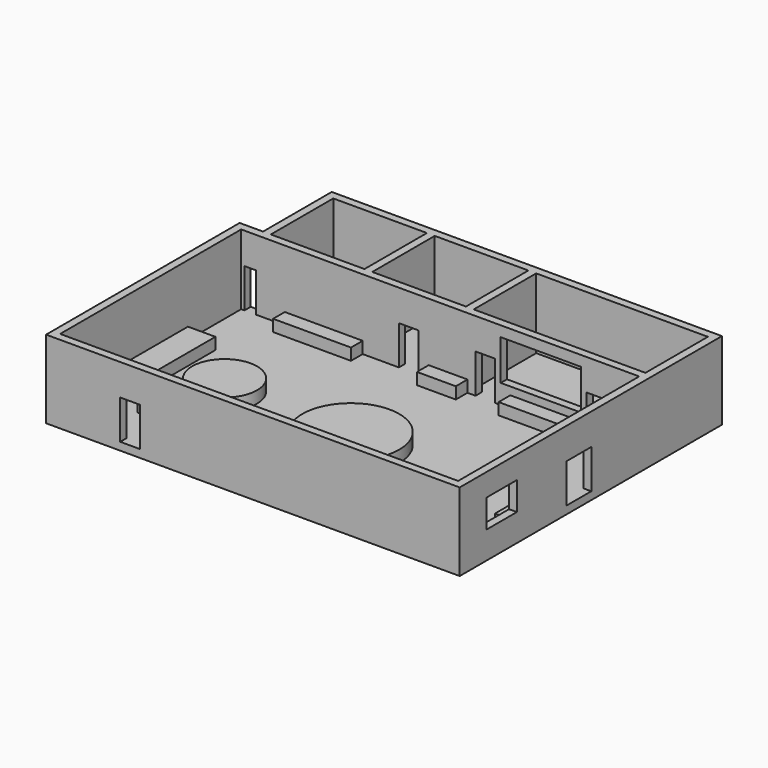
from build123d import *

# Parameters (mm, degrees)
F0_W      = 1346.2
F0_H      = 787.4
F1_DEPTH  = 254
F2_T      = -25.4
F3_W      = 1270
F3_H      = 254
F4_DEPTH  = 279.4
F5_T      = -25.4
F6_W      = 25.4
F6_H      = 254
F7_DEPTH  = 228.6
F8_W      = 63.5
F8_H      = 127
F9_DEPTH  = 25.4
F10_W     = 25.4
F10_H     = 254
F11_DEPTH = 228.6
F12_W     = 63.5
F12_H     = 127
F13_DEPTH = 25.4
F14_W     = 63.5
F14_H     = 127
F15_DEPTH = 25.4
F16_W     = 63.5
F16_H     = 127
F17_DEPTH = 25.4
F18_W     = 101.6
F18_H     = 127
F19_DEPTH = 25.4
F20_W     = 260.761320591
F20_H     = 131.0430763721
F21_DEPTH = 25.4
F22_W     = 124.2034286261
F22_H     = 91.7437373161
F23_DEPTH = 25.4
F24_W     = 38.1
F24_H     = 127
F25_DEPTH = 25.4
F26_W     = 43.4030661404
F26_H     = 204.1662087968
F27_DEPTH = 38.1
F28_W     = 217.1396613121
F28_H     = 47.6633155483
F29_DEPTH = 38.1
F30_W     = 126.3566912651
F30_H     = 47.6633155483
F31_DEPTH = 38.1
F32_W     = 253.5540759563
F32_H     = 47.6633155483
F33_DEPTH = 38.1
F34_W     = 206.0110867023
F34_H     = 100.5776971579
F35_DEPTH = 38.1
F36_W     = 89.4355172336
F36_H     = 266.5195167065
F37_DEPTH = 38.1
F38_R     = 105.778257903
F39_DEPTH = 38.1
F40_R     = 157.6742046587
F41_DEPTH = 38.1


# Not quite as in the source:
# - a shell that OpenCascade refuses in one call is made with other operations: the cavity is built on its own and cut out


with BuildPart() as f1:
    # F0 (on Top) → F1 (new body)
    with BuildSketch(Plane.XY):
        with Locations((-0.1443736255, 12.1287457604)):
            Rectangle(F0_W, F0_H)
    extrude(amount=F1_DEPTH)

    # F2
    f2_openings = [f1.faces().sort_by_distance(p)[0] for p in [
        (-0.144374, 12.128746, 254),
    ]]
    offset(amount=F2_T, openings=f2_openings)

    # F3 (on face) → F4 (join)
    with BuildSketch(Plane(origin=(0, 405.8287457604, 0), x_dir=(-1, 0, 0), z_dir=(0, 1, 0))):
        with Locations((-37.9556263745, 127)):
            Rectangle(F3_W, F3_H)
    extrude(amount=F4_DEPTH)

    # F5: a shell. OpenCascade refuses it in one call, so the cavity is built on its own and cut out:
    # the body offset inwards by the wall thickness, plus a prism from it out through each open face.
    f5_core = offset(f1.part, amount=F5_T, kind=Kind.INTERSECTION, mode=Mode.PRIVATE)
    f5_exits = [f5_core.faces().sort_by_distance(p)[0] for p in [
        (37.955626, 532.828746, 228.6),
    ]]
    add(f5_core, mode=Mode.SUBTRACT)
    extrude(f5_exits, amount=-F5_T, mode=Mode.SUBTRACT)

    # F6 (on face) → F7 (join)
    with BuildSketch(Plane.XY.offset(25.4)):
        with Locations((-254.1443736255, 532.8287457604)):
            Rectangle(F6_W, F6_H)
    extrude(amount=F7_DEPTH)

    # F8 (on face) → F9 (cut)
    with BuildSketch(Plane.YZ.offset(-241.4443736255)):
        with Locations((463.9602367878, 88.9)):
            Rectangle(F8_W, F8_H)
    extrude(amount=-F9_DEPTH, mode=Mode.SUBTRACT)

    # F10 (on face) → F11 (join)
    with BuildSketch(Plane.XY.offset(25.4)):
        with Locations((76.0556263745, 532.8287457604)):
            Rectangle(F10_W, F10_H)
    extrude(amount=F11_DEPTH)

    # F12 (on face) → F13 (cut)
    with BuildSketch(Plane.XZ.offset(-380.4287457604)):
        with Locations((-102.9241020679, 88.9)):
            Rectangle(F12_W, F12_H)
    extrude(amount=-F13_DEPTH, mode=Mode.SUBTRACT)

    # F14 (on face) → F15 (cut)
    with BuildSketch(Plane.XZ.offset(-380.4287457604)):
        with Locations((146.6235657334, 88.9)):
            Rectangle(F14_W, F14_H)
        with Locations((507.9058175087, 88.9)):
            Rectangle(F14_W, F14_H)
    extrude(amount=-F15_DEPTH, mode=Mode.SUBTRACT)

    # F16 (on face) → F17 (cut)
    with BuildSketch(Plane(origin=(0, -356.1712542396, 0), x_dir=(-1, 0, 0), z_dir=(0, 1, 0))):
        with Locations((400.1246755123, 88.9)):
            Rectangle(F16_W, F16_H)
    extrude(amount=-F17_DEPTH, mode=Mode.SUBTRACT)

    # F18 (on face) → F19 (cut)
    with BuildSketch(Plane(origin=(647.5556263745, 0, 0), x_dir=(0, -1, 0), z_dir=(-1, 0, 0))):
        with Locations((-102.9611633539, 88.9)):
            Rectangle(F18_W, F18_H)
    extrude(amount=-F19_DEPTH, mode=Mode.SUBTRACT)

    # F20 (on face) → F21 (cut)
    with BuildSketch(Plane.XZ.offset(-380.4287457604)):
        with Locations((327.1993100643, 154.4215381861)):
            Rectangle(F20_W, F20_H)
    extrude(amount=-F21_DEPTH, mode=Mode.SUBTRACT)

    # F22 (on face) → F23 (cut)
    with BuildSketch(Plane(origin=(647.5556263745, 0, 0), x_dir=(0, -1, 0), z_dir=(-1, 0, 0))):
        with Locations((211.2211957574, 134.7718686581)):
            Rectangle(F22_W, F22_H)
    extrude(amount=-F23_DEPTH, mode=Mode.SUBTRACT)

    # F24 (on face) → F25 (cut)
    with BuildSketch(Plane.XZ.offset(-380.4287457604)):
        with Locations((-618.1262156487, 88.9)):
            Rectangle(F24_W, F24_H)
    extrude(amount=-F25_DEPTH, mode=Mode.SUBTRACT)

    # F26 (on face) → F27 (join)
    with BuildSketch(Plane.XY.offset(25.4)):
        Polygon((647.5556263745, 380.4287457604), (539.6558175087, 380.4287457604), (539.6558175087, 332.765430212), (604.1525602341, 332.765430212), (604.1525602341, 209.5392942429), (647.5556263745, 209.5392942429), align=None)
        with Locations((625.8540933043, -49.9219410445)):
            Rectangle(F26_W, F26_H)
        Polygon((647.5556263745, -356.1712542396), (647.5556263745, -200.4013210535), (604.1525602341, -200.4013210535), (604.1525602341, -305.9601783752), (539.6558175087, -305.9601783752), (539.6558175087, -356.1712542396), align=None)
    extrude(amount=F27_DEPTH)

    # F28 (on face) → F29 (join)
    with BuildSketch(Plane.XY.offset(25.4)):
        with Locations((336.6870582104, 356.5970879862)):
            Rectangle(F28_W, F28_H)
    extrude(amount=F29_DEPTH)

    # F30 (on face) → F31 (join)
    with BuildSketch(Plane.XY.offset(25.4)):
        with Locations((25.5772807419, 356.5970879862)):
            Rectangle(F30_W, F30_H)
    extrude(amount=F31_DEPTH)

    # F32 (on face) → F33 (join)
    with BuildSketch(Plane.XY.offset(25.4)):
        with Locations((-379.1270405054, 356.5970879862)):
            Rectangle(F32_W, F32_H)
    extrude(amount=F33_DEPTH)

    # F34 (on face) → F35 (join)
    with BuildSketch(Plane.XY.offset(25.4)):
        with Locations((-395.1756507158, -178.2315000892)):
            Rectangle(F34_W, F34_H)
    extrude(amount=F35_DEPTH)

    # F36 (on face) → F37 (join)
    with BuildSketch(Plane.XY.offset(25.4)):
        with Locations((-603.1266150087, 30.4604619741)):
            Rectangle(F36_W, F36_H)
    extrude(amount=F37_DEPTH)

    # F38 (on face) → F39 (join)
    with BuildSketch(Plane.XY.offset(25.4)):
        with Locations((-397.5111842155, 0)):
            Circle(F38_R)
    extrude(amount=F39_DEPTH)

    # F40 (on face) → F41 (join)
    with BuildSketch(Plane.XY.offset(25.4)):
        with Locations((36.9560047984, -29.6728350222)):
            Circle(F40_R)
    extrude(amount=F41_DEPTH)


solid = f1.part
